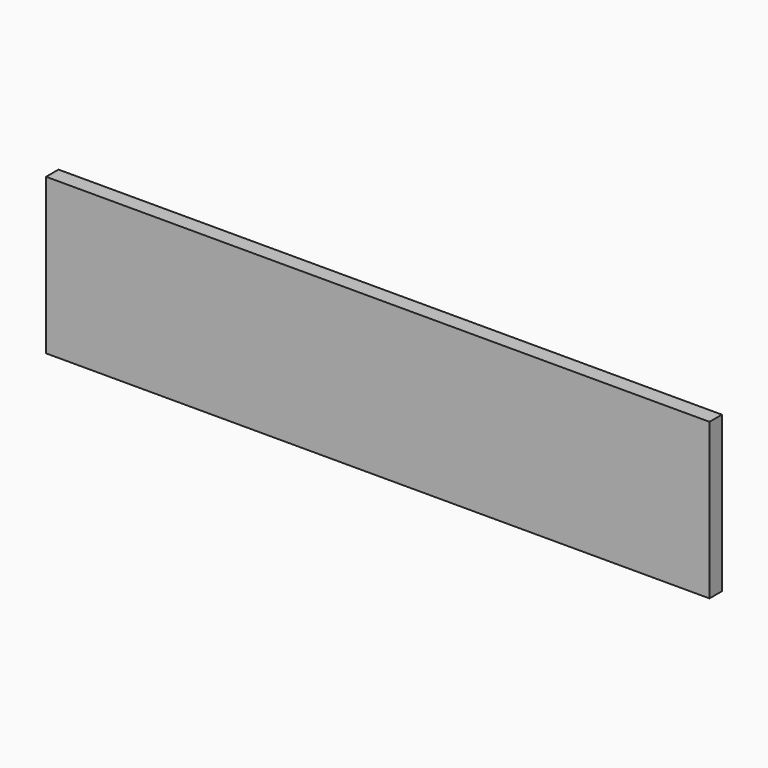
from build123d import *

# Parameters (mm, degrees)
F0_W     = 812.8
F0_H     = 190.5
F1_DEPTH = 19.05


# Not quite as in the source:
# - a feature names something its author has since deleted; it is built from what else it names


with BuildPart() as f1:
    # F0 (on Front) → F1 (new body)
    with BuildSketch(Plane.XZ):
        with Locations((406.4, 95.25)):
            Rectangle(F0_W, F0_H)
    extrude(amount=-F1_DEPTH)


solid = f1.part
